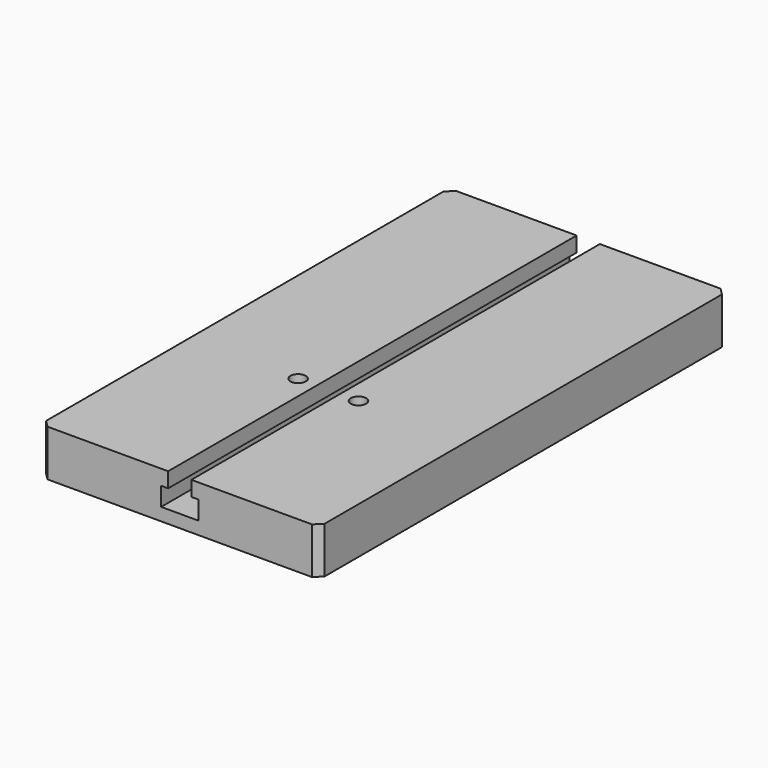
from build123d import *

# Parameters (mm, degrees)
F0_W           = 120
F0_H           = 220
F1_DEPTH       = 10
F3_DEPTH       = 220.001
F4_SIZE        = 3
F6_D           = 6.6
F6_CBORE_D     = 13
F6_CBORE_DEPTH = 4.6


# Not quite as in the source:
# - a pattern or mirror of a feature is missing from the dataset's text; its kind, count and spacing are read off the source's solid


with BuildPart() as f1:
    # F0 (on Top) → F1 (new body, symmetric)
    with BuildSketch(Plane.XY):
        Rectangle(F0_W, F0_H)
    extrude(amount=F1_DEPTH, both=True)

    # F2 (on face) → F3 (cut, through all)
    with BuildSketch(Plane.XZ.offset(110)):
        Polygon((5, 10), (-5, 10), (-5, 3.5), (-8, 3.5), (-8, -4.5), (8, -4.5), (8, 3.5), (5, 3.5), align=None)
    extrude(amount=-F3_DEPTH, mode=Mode.SUBTRACT)

    # F4
    f4_edges = [f1.edges().sort_by_distance(p)[0] for p in [
        (60, -110, 0),
        (60, 110, 0),
        (-60, 110, 0),
        (-60, -110, 0),
    ]]
    chamfer(f4_edges, length=F4_SIZE)

    # F6 (through all)
    with Locations(Plane(origin=(0, 0, -10), x_dir=(1, 0, 0), z_dir=(0, 0, -1))):
        with Locations((-13, 30)):
            f6 = CounterBoreHole(F6_D / 2, F6_CBORE_D / 2, F6_CBORE_DEPTH)

    # F6_copies: F6 across plane
    add(f6.mirror(Plane(origin=(0, 0, 0), x_dir=(0, 0, 1), z_dir=(1, 0, 0))), mode=Mode.SUBTRACT)


solid = f1.part
